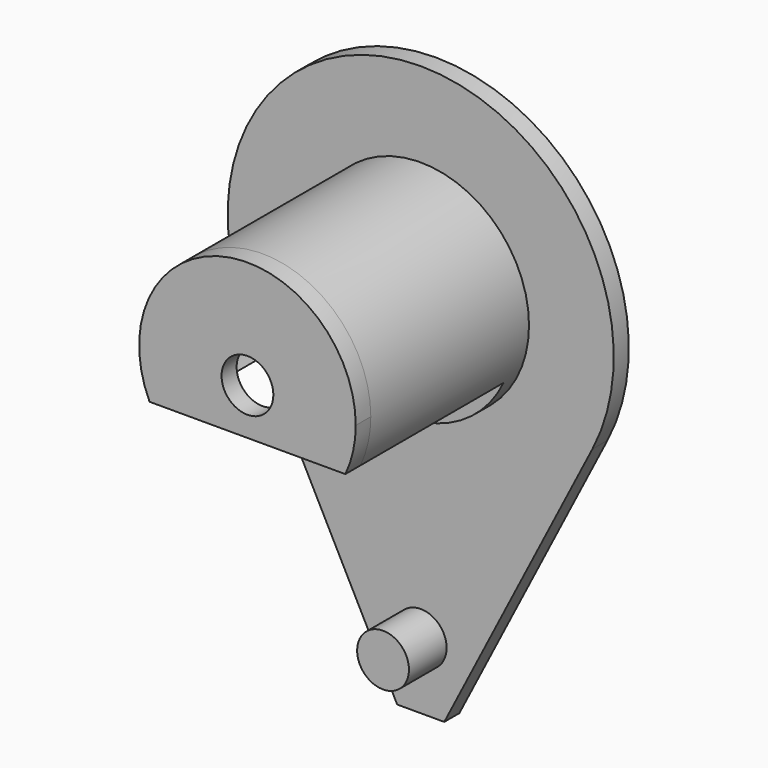
from build123d import *

# Parameters (mm, degrees)
F0_R      = 2.75
F0_R_2    = 11.5
F1_DEPTH  = 2
F3_DEPTH  = 29
F4_R      = 11.5
F4_R_2    = 2.75
F5_DEPTH  = 2
F0_R_3    = 9.5
F8_DEPTH  = 23
F9_DEPTH  = 7
F11_DEPTH = 19
F12_R     = 2.75
F13_DEPTH = 2


with BuildPart() as f1:
    # F0 (on Front) → F1 (new body)
    with BuildSketch(Plane.XZ):
        with BuildLine():
            Line((2.5, -40), (18.2350646454, -9.3665584597))
            ThreePointArc((18.2350646454, -9.3665584597), (0, 20.5), (-18.2350646454, -9.3665584597))
            Line((-18.2350646454, -9.3665584597), (-2.5, -40))
            Line((-2.5, -40), (2.5, -40))
        make_face()
        with Locations((0, -33)):
            Circle(F0_R, mode=Mode.SUBTRACT)
        Circle(F0_R_2, mode=Mode.SUBTRACT)
    extrude(amount=F1_DEPTH)

    # F0 (on Front) → F8 (join)
    with BuildSketch(Plane.XZ):
        Circle(F0_R_2)
        Circle(F0_R_3, mode=Mode.SUBTRACT)
    extrude(amount=F8_DEPTH)

    # F0 (on Front) → F9 (join)
    with BuildSketch(Plane.XZ):
        with Locations((0, -33)):
            Circle(F0_R)
    extrude(amount=F9_DEPTH)

    # F10 (on face) → F11 (cut)
    with BuildSketch(Plane.XZ.offset(23)):
        with BuildLine():
            Line((-8.129197368, -4.9159078665), (-10.3963382904, -4.9159078665))
            ThreePointArc((-10.3963382904, -4.9159078665), (0, -11.5), (10.3963382904, -4.9159078665))
            Line((10.3963382904, -4.9159078665), (8.129197368, -4.9159078665))
            ThreePointArc((8.129197368, -4.9159078665), (0, -9.5), (-8.129197368, -4.9159078665))
        make_face()
    extrude(amount=-F11_DEPTH, mode=Mode.SUBTRACT)

    # F12 (on face) → F13 (join)
    with BuildSketch(Plane.XZ.offset(23)):
        with BuildLine():
            Line((8.129197368, -4.9159078665), (10.3963382904, -4.9159078665))
            ThreePointArc((10.3963382904, -4.9159078665), (11.2206927224, -2.5191377156), (11.5, 0))
            ThreePointArc((11.5, 0), (-2.5191377156, 11.2206927224), (-10.3963382904, -4.9159078665))
            Line((-10.3963382904, -4.9159078665), (-8.129197368, -4.9159078665))
            ThreePointArc((-8.129197368, -4.9159078665), (-2.5517273565, 9.15088452), (9.5, 0))
            ThreePointArc((9.5, 0), (9.15088452, -2.5517273565), (8.129197368, -4.9159078665))
        make_face()
        with BuildLine():
            Line((-8.129197368, -4.9159078665), (8.129197368, -4.9159078665))
            ThreePointArc((8.129197368, -4.9159078665), (9.15088452, -2.5517273565), (9.5, 0))
            ThreePointArc((9.5, 0), (-2.5517273565, 9.15088452), (-8.129197368, -4.9159078665))
        make_face()
        Circle(F12_R, mode=Mode.SUBTRACT)
    extrude(amount=F13_DEPTH)


with BuildPart() as f3:
    # F2 (on face) → F3 (new body)
    with BuildSketch(Plane(origin=(0, 0, 0), x_dir=(-1, 0, 0), z_dir=(0, 1, 0))):
        with BuildLine():
            ThreePointArc((0, 11.5), (-8.1317279836, 8.1317279836), (-11.5, 0))
            ThreePointArc((-11.5, 0), (-11.2103927734, -2.5645845405), (-10.3561575886, -5))
            Line((-10.3561575886, -5), (-8.6602540378, -5))
            ThreePointArc((-8.6602540378, -5), (0, 10), (8.6602540378, -5))
            Line((8.6602540378, -5), (10.3561575886, -5))
            ThreePointArc((10.3561575886, -5), (11.2103927734, -2.5645845405), (11.5, 0))
            ThreePointArc((11.5, 0), (8.1317279836, 8.1317279836), (0, 11.5))
        make_face()
    extrude(amount=F3_DEPTH)


with BuildPart() as f5:
    # F4 (on Front) → F5 (new body)
    with BuildSketch(Plane.XZ):
        Circle(F4_R)
        Circle(F4_R_2, mode=Mode.SUBTRACT)
    extrude(amount=F5_DEPTH)


solid = f1.part
